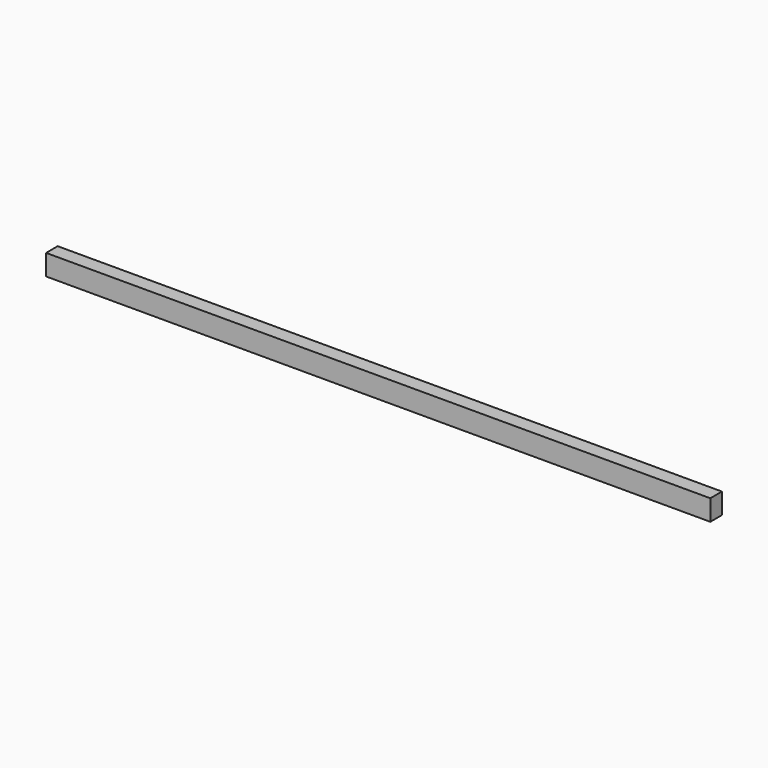
from build123d import *

# Parameters (mm, degrees)
F1_W     = 44.45
F1_H     = 63.5
F2_DEPTH = 2032


# Not quite as in the source:
# - a variable given as a bare number and used for a length is read in inches; the dataset says mm whatever the document's units were


with BuildPart() as f2:
    # F1 (on Right) → F2 (new body)
    with BuildSketch(Plane.YZ):
        with Locations((-22.225, 31.75)):
            Rectangle(F1_W, F1_H)
    extrude(amount=F2_DEPTH)


solid = f2.part
